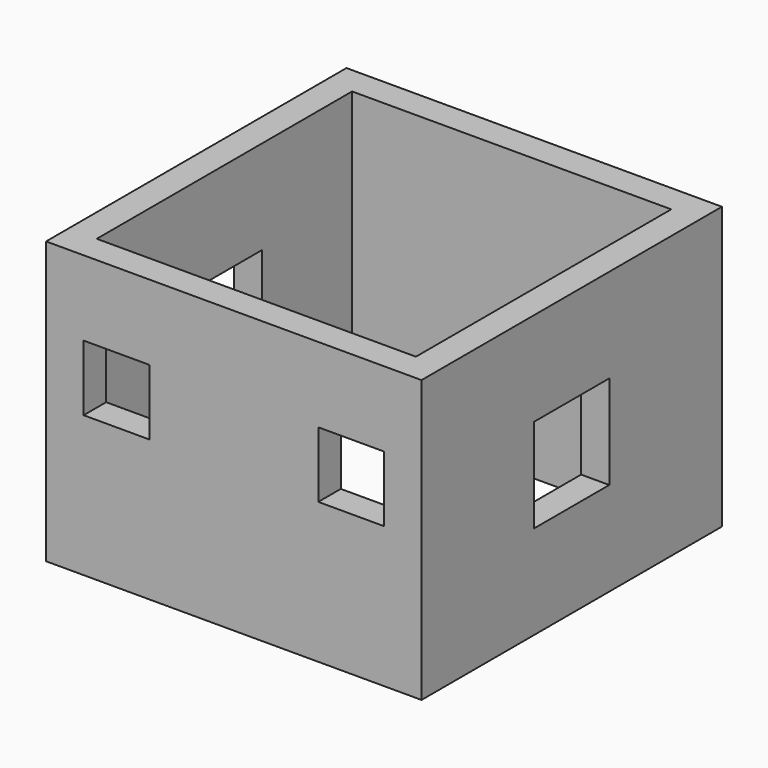
from build123d import *

# Parameters (mm, degrees)
F0_W      = 50.8
F0_H      = 50.8
F1_DEPTH  = 38.1
F2_T      = -3.81
F10_W     = 12.7
F10_H     = 12.7
F11_DEPTH = 25.4
F12_W     = 12.7
F12_H     = 12.7
F13_DEPTH = 25.4
F14_W     = 8.89
F14_H     = 8.89
F15_DEPTH = 25.4


# Not quite as in the source:
# - the program builds the solid bodies; features that only make, move or delete a surface that nothing else refers to are left out


with BuildPart() as f1:
    # F0 (on Top) → F1 (new body)
    with BuildSketch(Plane.XY):
        with Locations((0.1272018999, -1.6994403997)):
            Rectangle(F0_W, F0_H)
    extrude(amount=F1_DEPTH)

    # F2
    f2_openings = [f1.faces().sort_by_distance(p)[0] for p in [
        (0.127202, -1.69944, 38.1),
        (0.127202, -1.69944, 0),
    ]]
    offset(amount=F2_T, openings=f2_openings)

    # F10 (on face) → F11 (cut)
    with BuildSketch(Plane.YZ.offset(25.5272018999)):
        with Locations((-1.6994403997, 19.05)):
            Rectangle(F10_W, F10_H)
    extrude(amount=-F11_DEPTH, mode=Mode.SUBTRACT)

    # F12 (on face) → F13 (cut)
    with BuildSketch(Plane(origin=(-25.2727981001, 0, 0), x_dir=(0, -1, 0), z_dir=(-1, 0, 0))):
        with Locations((1.6994403997, 19.05)):
            Rectangle(F12_W, F12_H)
    extrude(amount=-F13_DEPTH, mode=Mode.SUBTRACT)

    # F14 (on face) → F15 (cut)
    with BuildSketch(Plane.XZ.offset(27.0994403997)):
        with Locations((16.0022018999, 23.495)):
            Rectangle(F14_W, F14_H)
        with Locations((-15.7477981001, 23.495)):
            Rectangle(F14_W, F14_H)
    extrude(amount=-F15_DEPTH, mode=Mode.SUBTRACT)


solid = f1.part
